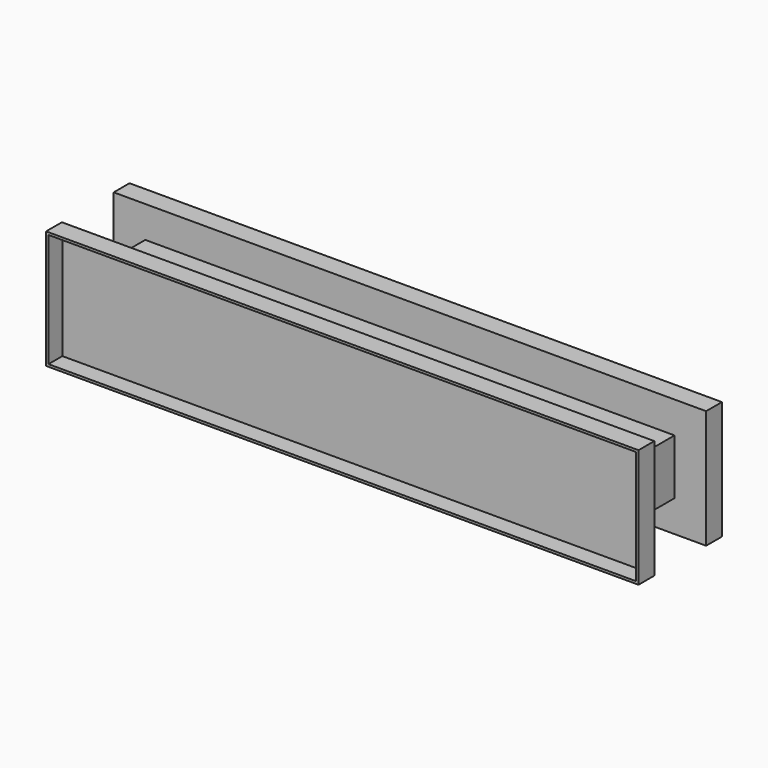
from build123d import *

# Parameters (mm, degrees)
F0_W     = 25
F0_H     = 150
F1_DEPTH = 375
F2_T     = -3
F4_DEPTH = 335
F5_W     = 35
F5_H     = 70
F6_DEPTH = 3


# Not quite as in the source:
# - a pattern or mirror of a feature is missing from the dataset's text; its kind, count and spacing are read off the source's solid


with BuildPart() as f1:
    # F0 (on Right) → F1 (new body, symmetric)
    with BuildSketch(Plane.YZ):
        with Locations((53.5, 0)):
            Rectangle(F0_W, F0_H)
    extrude(amount=F1_DEPTH, both=True)

    # F2
    f2_openings = [f1.faces().sort_by_distance(p)[0] for p in [
        (0, 66, 0),
    ]]
    offset(amount=F2_T, openings=f2_openings)

    # F3 (on Right) → F4 (join, symmetric)
    with BuildSketch(Plane.YZ):
        Polygon((41, 32), (41, 35), (6, 35), (6, 15), (9, 15), (9, 32), align=None)
        Polygon((6, -35), (41, -35), (41, -32), (9, -32), (9, -15), (6, -15), align=None)
    extrude(amount=F4_DEPTH, both=True)

    # F5 (on face) → F6 (join)
    with BuildSketch(Plane.YZ.offset(335)):
        with Locations((23.5, 0)):
            Rectangle(F5_W, F5_H)
    f6 = extrude(amount=-F6_DEPTH)

    # F6_copies: F6 across plane
    add(f6.mirror(Plane(origin=(0, 0, 0), x_dir=(0, 0, -1), z_dir=(-1, 0, 0))))


with BuildPart() as f7_1:
    # F7: instance of F1
    add(f1.part.mirror(Plane.XZ))


solid = Compound([f1.part, f7_1.part])
